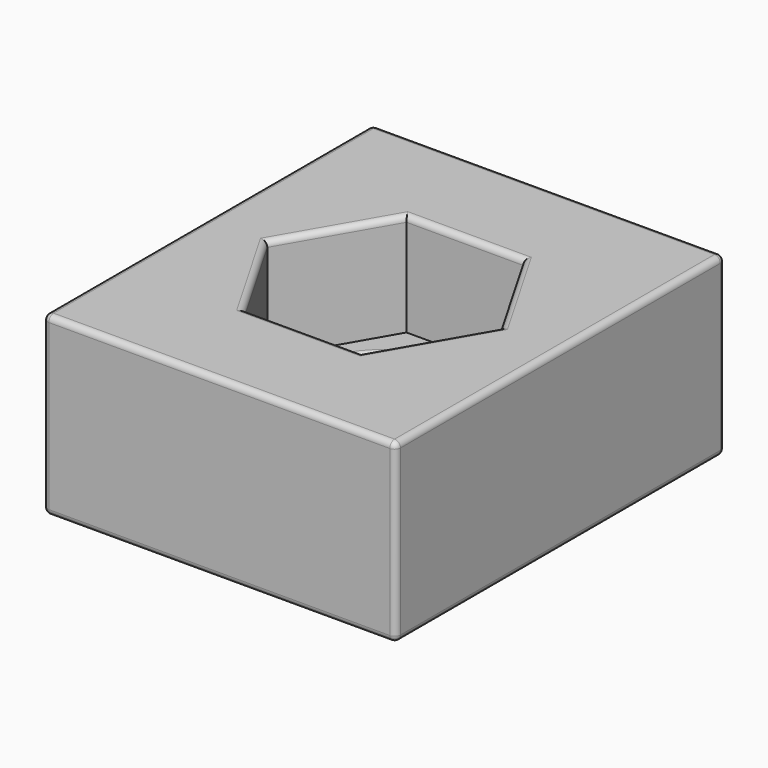
from build123d import *

# Parameters (mm, degrees)
F4_W         = 12
F4_H         = 14
F4_R         = 2.75
F0_DEPTH     = 6
F5_DEPTH     = 3.5
F2_R         = 0.2
F3_T1_DEPTH  = 13.6
F3_S5_W      = 0.2
F3_S5_H      = 0.2
F3_T6_DEPTH  = 0.2
F3_S11_W     = 0.2
F3_S11_H     = 0.2
F3_T12_DEPTH = 0.2


# Not quite as in the source:
# - a fillet or chamfer that OpenCascade refuses, or shapes differently, is made with other operations: its cross-section is extruded or revolved along the edge and cut away or added


with BuildPart() as f0:
    # F4 (on Top) → F0 (new body)
    with BuildSketch(Plane.XY):
        with Locations((6, 2.0147956188)):
            Rectangle(F4_W, F4_H)
        with Locations((6, 2.0147956188)):
            Circle(F4_R, mode=Mode.SUBTRACT)
    extrude(amount=F0_DEPTH)

    # F1 (on face) → F5 (cut)
    with BuildSketch(Plane.XY.offset(6)):
        Polygon((4.015, -1.4233252342), (7.985, -1.4233252342), (9.97, 2.0147956188), (7.985, 5.4529164718), (4.015, 5.4529164718), (2.03, 2.0147956188), align=None)
    extrude(amount=-F5_DEPTH, mode=Mode.SUBTRACT)

    # F2
    f2_edges = [f0.edges().sort_by_distance(p)[0] for p in [
        (6, -4.985204, 6),
        (0, 2.014796, 6),
        (6, 9.014796, 6),
        (12, 2.014796, 6),
        (6, 5.452916, 6),
        (8.9775, 3.733856, 6),
        (8.9775, 0.295735, 6),
        (6, -1.423325, 6),
        (3.0225, 0.295735, 6),
        (3.0225, 3.733856, 6),
        (3.25, 2.014796, 2.5),
        (12, -4.985204, 3),
        (12, 9.014796, 3),
        (12, 2.014796, 0),
        (6, -4.985204, 0),
        (0, -4.985204, 3),
        (3.25, 2.014796, 0),
        (6, 9.014796, 0),
        (0, 9.014796, 3),
    ]]
    fillet(f2_edges, radius=F2_R)

    # F3: fillet of radius 0.2 on 1 edges, made by hand

    # F3_s2 → F3_t1 (cut)
    with BuildSketch(Plane.XZ.offset(-8.8147956188)):
        with BuildLine():
            ThreePointArc((0, 0.2), (0.0585786438, 0.0585786438), (0.2, 0))
            Line((0.2, 0), (0, 0))
            Line((0, 0), (0, 0.2))
        make_face()
    extrude(amount=F3_T1_DEPTH, mode=Mode.SUBTRACT)


with BuildPart() as f3_tool4:
    # F3_s5 → F3_t6 (new body)
    with BuildSketch(Plane.YZ.offset(0.2)):
        with Locations((8.9147956188, 0.1)):
            Rectangle(F3_S5_W, F3_S5_H)
    extrude(amount=-F3_T6_DEPTH)

    # F3_s7 → F3_t8 (revolve, cut)
    with BuildSketch(Plane(origin=(0.2, 8.8147956188, 0.2), x_dir=(0, -0.7071067812, 0.7071067812), z_dir=(0, -0.7071067812, -0.7071067812))):
        with BuildLine():
            ThreePointArc((0, -0.2), (0.2, 0), (0, 0.2))
            Line((0, 0.2), (0, -0.2))
        make_face()
    revolve(axis=Axis((0.2, 8.8147956188, 0.2), (-1, 0, 0)), mode=Mode.SUBTRACT)


with BuildPart() as f0_1:
    add(f0.part)

    # F3_t3: cut F3_tool4
    add(f3_tool4.part, mode=Mode.SUBTRACT)


with BuildPart() as f3_tool10:
    # F3_s11 → F3_t12 (new body)
    with BuildSketch(Plane.YZ.offset(0.2)):
        with Locations((-4.8852043812, 0.1)):
            Rectangle(F3_S11_W, F3_S11_H)
    extrude(amount=-F3_T12_DEPTH)

    # F3_s13 → F3_t14 (revolve, cut)
    with BuildSketch(Plane(origin=(0.2, -4.7852043812, 0.2), x_dir=(0, 0.7071067812, 0.7071067812), z_dir=(0, -0.7071067812, 0.7071067812))):
        with BuildLine():
            ThreePointArc((0, -0.2), (0.2, 0), (0, 0.2))
            Line((0, 0.2), (0, -0.2))
        make_face()
    revolve(axis=Axis((0.2, -4.7852043812, 0.2), (-1, 0, 0)), mode=Mode.SUBTRACT)


with BuildPart() as f0_2:
    add(f0_1.part)

    # F3_t9: cut F3_tool10
    add(f3_tool10.part, mode=Mode.SUBTRACT)


solid = f0_2.part
